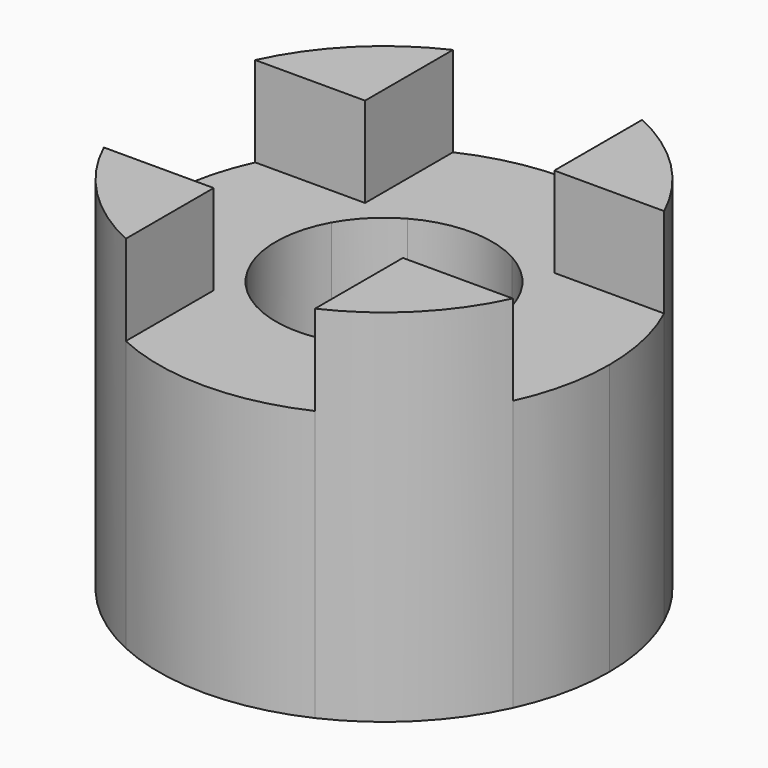
from build123d import *

# Parameters (mm, degrees)
F1_DEPTH = 15
F2_DEPTH = 20
F0_R     = 3.5
F3_DEPTH = 3


with BuildPart() as f1:
    # F0 (on Top) → F1 (new body)
    with BuildSketch(Plane.XY):
        with BuildLine():
            Line((5.25, 5.25), (11.3440513045, 5.25))
            ThreePointArc((11.3440513045, 5.25), (8.8388347648, 8.8388347648), (5.25, 11.3440513045))
            Line((5.25, 11.3440513045), (5.25, 5.25))
        make_face()
        with BuildLine():
            Line((5.25, 5.25), (5.25, 11.3440513045))
            ThreePointArc((5.25, 11.3440513045), (0, 12.5), (-5.25, 11.3440513045))
            Line((-5.25, 11.3440513045), (-5.25, 5.25))
            Line((-5.25, 5.25), (-2.9047375097, 5.25))
            ThreePointArc((-2.9047375097, 5.25), (0, 6), (2.9047375097, 5.25))
            Line((2.9047375097, 5.25), (5.25, 5.25))
        make_face()
        with BuildLine():
            Line((-5.25, 5.25), (-5.25, 11.3440513045))
            ThreePointArc((-5.25, 11.3440513045), (-8.8388347648, 8.8388347648), (-11.3440513045, 5.25))
            Line((-11.3440513045, 5.25), (-5.25, 5.25))
        make_face()
        with BuildLine():
            Line((-5.25, 5.25), (-11.3440513045, 5.25))
            ThreePointArc((-11.3440513045, 5.25), (-12.5, 0), (-11.3440513045, -5.25))
            Line((-11.3440513045, -5.25), (-5.25, -5.25))
            Line((-5.25, -5.25), (-5.25, -2.9047375097))
            ThreePointArc((-5.25, -2.9047375097), (-6, 0), (-5.25, 2.9047375097))
            Line((-5.25, 2.9047375097), (-5.25, 5.25))
        make_face()
        with BuildLine():
            ThreePointArc((-11.3440513045, -5.25), (-8.8388347648, -8.8388347648), (-5.25, -11.3440513045))
            Line((-5.25, -11.3440513045), (-5.25, -5.25))
            Line((-5.25, -5.25), (-11.3440513045, -5.25))
        make_face()
        with BuildLine():
            ThreePointArc((-5.25, -11.3440513045), (0, -12.5), (5.25, -11.3440513045))
            Line((5.25, -11.3440513045), (5.25, -5.25))
            Line((5.25, -5.25), (2.9047375097, -5.25))
            ThreePointArc((2.9047375097, -5.25), (0, -6), (-2.9047375097, -5.25))
            Line((-2.9047375097, -5.25), (-5.25, -5.25))
            Line((-5.25, -5.25), (-5.25, -11.3440513045))
        make_face()
        with BuildLine():
            ThreePointArc((5.25, -11.3440513045), (8.8388347648, -8.8388347648), (11.3440513045, -5.25))
            Line((11.3440513045, -5.25), (5.25, -5.25))
            Line((5.25, -5.25), (5.25, -11.3440513045))
        make_face()
        with BuildLine():
            ThreePointArc((11.3440513045, -5.25), (12.207592746, -2.6878763637), (12.5, 0))
            ThreePointArc((12.5, 0), (12.207592746, 2.6878763637), (11.3440513045, 5.25))
            Line((11.3440513045, 5.25), (5.25, 5.25))
            Line((5.25, 5.25), (5.25, 2.9047375097))
            ThreePointArc((5.25, 2.9047375097), (5.8094750193, 1.5), (6, 0))
            ThreePointArc((6, 0), (5.8094750193, -1.5), (5.25, -2.9047375097))
            Line((5.25, -2.9047375097), (5.25, -5.25))
            Line((5.25, -5.25), (11.3440513045, -5.25))
        make_face()
        with BuildLine():
            Line((5.25, 2.9047375097), (5.25, 5.25))
            Line((5.25, 5.25), (2.9047375097, 5.25))
            ThreePointArc((2.9047375097, 5.25), (4.2426406871, 4.2426406871), (5.25, 2.9047375097))
        make_face()
        with BuildLine():
            Line((-2.9047375097, 5.25), (-5.25, 5.25))
            Line((-5.25, 5.25), (-5.25, 2.9047375097))
            ThreePointArc((-5.25, 2.9047375097), (-4.2426406871, 4.2426406871), (-2.9047375097, 5.25))
        make_face()
        with BuildLine():
            Line((-5.25, -2.9047375097), (-5.25, -5.25))
            Line((-5.25, -5.25), (-2.9047375097, -5.25))
            ThreePointArc((-2.9047375097, -5.25), (-4.2426406871, -4.2426406871), (-5.25, -2.9047375097))
        make_face()
        with BuildLine():
            Line((2.9047375097, -5.25), (5.25, -5.25))
            Line((5.25, -5.25), (5.25, -2.9047375097))
            ThreePointArc((5.25, -2.9047375097), (4.2426406871, -4.2426406871), (2.9047375097, -5.25))
        make_face()
    extrude(amount=F1_DEPTH)

    # F0 (on Top) → F3 (join)
    with BuildSketch(Plane.XY):
        with BuildLine():
            Line((5.25, -2.9047375097), (5.25, 2.9047375097))
            ThreePointArc((5.25, 2.9047375097), (4.2426406871, 4.2426406871), (2.9047375097, 5.25))
            Line((2.9047375097, 5.25), (-2.9047375097, 5.25))
            ThreePointArc((-2.9047375097, 5.25), (-4.2426406871, 4.2426406871), (-5.25, 2.9047375097))
            Line((-5.25, 2.9047375097), (-5.25, -2.9047375097))
            ThreePointArc((-5.25, -2.9047375097), (-4.2426406871, -4.2426406871), (-2.9047375097, -5.25))
            Line((-2.9047375097, -5.25), (2.9047375097, -5.25))
            ThreePointArc((2.9047375097, -5.25), (4.2426406871, -4.2426406871), (5.25, -2.9047375097))
        make_face()
        Circle(F0_R, mode=Mode.SUBTRACT)
        with BuildLine():
            Line((-2.9047375097, 5.25), (2.9047375097, 5.25))
            ThreePointArc((2.9047375097, 5.25), (0, 6), (-2.9047375097, 5.25))
        make_face()
        with BuildLine():
            Line((-5.25, -2.9047375097), (-5.25, 2.9047375097))
            ThreePointArc((-5.25, 2.9047375097), (-6, 0), (-5.25, -2.9047375097))
        make_face()
        with BuildLine():
            ThreePointArc((-2.9047375097, -5.25), (0, -6), (2.9047375097, -5.25))
            Line((2.9047375097, -5.25), (-2.9047375097, -5.25))
        make_face()
        with BuildLine():
            ThreePointArc((6, 0), (5.8094750193, 1.5), (5.25, 2.9047375097))
            Line((5.25, 2.9047375097), (5.25, -2.9047375097))
            ThreePointArc((5.25, -2.9047375097), (5.8094750193, -1.5), (6, 0))
        make_face()
    extrude(amount=F3_DEPTH)


with BuildPart() as f2:
    # F0 (on Top) → F2 (new body)
    with BuildSketch(Plane.XY):
        with BuildLine():
            Line((5.25, 5.25), (11.3440513045, 5.25))
            ThreePointArc((11.3440513045, 5.25), (8.8388347648, 8.8388347648), (5.25, 11.3440513045))
            Line((5.25, 11.3440513045), (5.25, 5.25))
        make_face()
    extrude(amount=F2_DEPTH)


with BuildPart() as f2b:
    # F0 (on Top) → F2, piece 2 (new body)
    with BuildSketch(Plane.XY):
        with BuildLine():
            ThreePointArc((5.25, -11.3440513045), (8.8388347648, -8.8388347648), (11.3440513045, -5.25))
            Line((11.3440513045, -5.25), (5.25, -5.25))
            Line((5.25, -5.25), (5.25, -11.3440513045))
        make_face()
    extrude(amount=F2_DEPTH)


with BuildPart() as f2c:
    # F0 (on Top) → F2, piece 3 (new body)
    with BuildSketch(Plane.XY):
        with BuildLine():
            Line((-5.25, 5.25), (-5.25, 11.3440513045))
            ThreePointArc((-5.25, 11.3440513045), (-8.8388347648, 8.8388347648), (-11.3440513045, 5.25))
            Line((-11.3440513045, 5.25), (-5.25, 5.25))
        make_face()
    extrude(amount=F2_DEPTH)


with BuildPart() as f2d:
    # F0 (on Top) → F2, piece 4 (new body)
    with BuildSketch(Plane.XY):
        with BuildLine():
            ThreePointArc((-11.3440513045, -5.25), (-8.8388347648, -8.8388347648), (-5.25, -11.3440513045))
            Line((-5.25, -11.3440513045), (-5.25, -5.25))
            Line((-5.25, -5.25), (-11.3440513045, -5.25))
        make_face()
    extrude(amount=F2_DEPTH)


solid = Compound([f1.part, f2.part, f2b.part, f2c.part, f2d.part])
